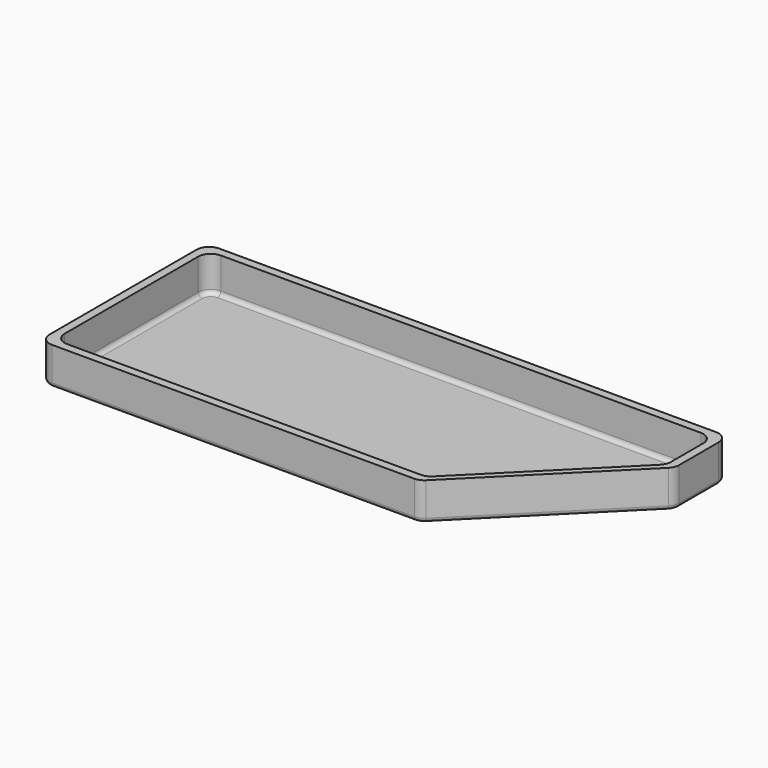
from build123d import *

# Parameters (mm, degrees)
F1_DEPTH = 9
F3_DEPTH = 8.5
F4_R     = 3
F5_R     = 1


# Not quite as in the source:
# - a feature names something its author has since deleted; it is built from what else it names


with BuildPart() as f1:
    # F0 (on Top) → F1 (new body)
    with BuildSketch(Plane.XY):
        Polygon((-62.5, -25), (28.5, -25), (62.5, 9), (62.5, 25), (-62.5, 25), align=None)
    extrude(amount=F1_DEPTH)

    # F2 (on face) → F3 (cut)
    with BuildSketch(Plane.XY.offset(9)):
        Polygon((60.5, 9), (60.5, 23), (-60.5, 23), (-60.5, -23), (28.5, -23), align=None)
    extrude(amount=-F3_DEPTH, mode=Mode.SUBTRACT)

    # F4
    f4_edges = [f1.edges().sort_by_distance(p)[0] for p in [
        (-60.5, 23, 4.75),
        (60.5, 23, 4.75),
        (60.5, 9, 4.75),
        (28.5, -23, 4.75),
        (-60.5, -23, 4.75),
        (62.5, 25, 4.5),
        (62.5, 9, 4.5),
        (28.5, -25, 4.5),
        (-62.5, 25, 4.5),
        (-62.5, -25, 4.5),
    ]]
    fillet(f4_edges, radius=F4_R)

    # F5
    f5_edges = [f1.edges().sort_by_distance(p)[0] for p in [
        (60.5, 15.12132, 0.5),
        (60.271639, 9.09459, 0.5),
        (59.62132, 22.12132, 0.5),
        (44.5, -7, 0.5),
        (0, 23, 0.5),
        (28.40541, -22.771639, 0.5),
        (-59.62132, 22.12132, 0.5),
        (-15.12132, -23, 0.5),
        (-60.5, 0, 0.5),
        (-59.62132, -22.12132, 0.5),
        (-16.12132, -25, 0),
        (-61.62132, -24.12132, 0),
        (28.40541, -24.771639, 0),
        (-62.5, 0, 0),
        (45.5, -8, 0),
        (-61.62132, 24.12132, 0),
        (62.271639, 9.09459, 0),
        (0, 25, 0),
        (62.5, 16.12132, 0),
        (61.62132, 24.12132, 0),
    ]]
    fillet(f5_edges, radius=F5_R)


solid = f1.part
